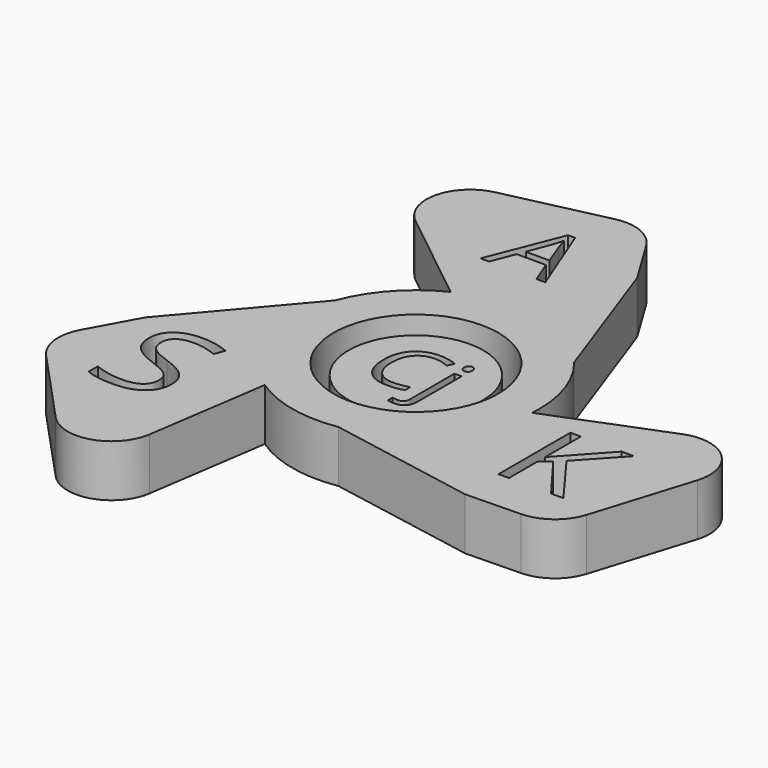
from build123d import *

# Parameters (mm, degrees)
F0_R          = 11.1
F1_DEPTH      = 7
F2_TEXT_SIZE  = 16.9441087766
F3_DEPTH      = 25.4
F4_TEXT_SIZE  = 13.7672423282
F5_DEPTH      = 25.4
F6_TEXT_SIZE  = 19.1516820431
F7_DEPTH      = 25.4
F8_R          = 9.0670245161
F9_DEPTH      = 5.588
F10_TEXT_SIZE = 11.9094963237
F11_DEPTH     = 25.4
F13_W         = 6
F13_H         = 1
F13_W_2       = 1
F13_H_2       = 3
F14_DEPTH     = 3


# Not quite as in the source:
# - Text() gives the source's letters only with a copy of the font that has no kerning and outlines rounded to 1/6400 em; it was checked with that copy


with BuildPart() as f1:
    # F0 (on Top) → F1 (new body)
    with BuildSketch(Plane.XY):
        with BuildLine():
            ThreePointArc((16.5940088671, -1.1747814046), (16.6251551137, -0.587757669), (16.635541519, 0))
            ThreePointArc((16.635541519, 0), (15.664947067, 5.5991673506), (12.8664216519, 10.5449720486))
            ThreePointArc((12.8664216519, 10.5449720486), (3.5598178716, 16.2501981019), (-7.2796138933, 14.9582239319))
            ThreePointArc((-7.2796138933, 14.9582239319), (-12.293175437, 11.2079917606), (-15.5654245023, 5.8701619821))
            ThreePointArc((-15.5654245023, 5.8701619821), (-15.8529933086, -5.0422063413), (-9.3143949738, -13.7834425273))
            ThreePointArc((-9.3143949738, -13.7834425273), (-3.5598178716, -16.2501981019), (2.6990028503, -16.4151340307))
            ThreePointArc((2.6990028503, -16.4151340307), (12.293175437, -11.2079917606), (16.5940088671, -1.1747814046))
        make_face()
        Circle(F0_R, mode=Mode.SUBTRACT)
        with BuildLine():
            ThreePointArc((-7.2796138933, 14.9582239319), (3.5598178716, 16.2501981019), (12.8664216519, 10.5449720486))
            Line((12.8664216519, 10.5449720486), (6.0360450298, 29.6823140234))
            Line((6.0360450298, 29.6823140234), (2.1992372512, 35.9986009481))
            ThreePointArc((2.1992372512, 35.9986009481), (-0.5333593719, 38.362277675), (-4.1319169388, 38.6854423552))
            Line((-4.1319169388, 38.6854423552), (-17.8556635882, 35.5845182616))
            ThreePointArc((-17.8556635882, 35.5845182616), (-22.2992502488, 31.1502452294), (-20.2187305905, 25.227435281))
            Line((-20.2187305905, 25.227435281), (-7.2796138933, 14.9582239319))
        make_face()
        with BuildLine():
            Line((31.9569651209, 4.8962166832), (16.5940088671, -1.1747814046))
            ThreePointArc((16.5940088671, -1.1747814046), (12.293175437, -11.2079917606), (2.6990028503, -16.4151340307))
            Line((2.6990028503, -16.4151340307), (22.6876154725, -20.0685253458))
            Line((22.6876154725, -20.0685253458), (30.0760842961, -19.9038958025))
            ThreePointArc((30.0760842961, -19.9038958025), (33.4893866995, -18.7192360721), (35.5685343057, -15.7643761422))
            Line((35.5685343057, -15.7643761422), (39.7449285901, -2.328800862))
            ThreePointArc((39.7449285901, -2.328800862), (38.1265288272, 3.7365945861), (31.9569651209, 4.8962166832))
        make_face()
        with BuildLine():
            ThreePointArc((-9.3143949738, -13.7834425273), (-15.8529933086, -5.0422063413), (-15.5654245023, 5.8701619821))
            Line((-15.5654245023, 5.8701619821), (-28.7236605022, -9.6137886775))
            Line((-28.7236605022, -9.6137886775), (-32.2753215473, -16.0947051456))
            ThreePointArc((-32.2753215473, -16.0947051456), (-32.9560273276, -19.6430416029), (-31.4366173668, -22.921066213))
            Line((-31.4366173668, -22.921066213), (-21.8892650019, -33.2557173997))
            ThreePointArc((-21.8892650019, -33.2557173997), (-15.8272785784, -34.8868398155), (-11.7382345304, -30.1236519642))
            Line((-11.7382345304, -30.1236519642), (-9.3143949738, -13.7834425273))
        make_face()
    extrude(amount=F1_DEPTH)

    # F2 (on face) → F3 (cut)
    with BuildSketch(Plane.XY.offset(7)):
        with Locations((20.8926647902, -14.2971209716)):
            Text('K', F2_TEXT_SIZE, font='Open Sans', text_align=(TextAlign.LEFT, TextAlign.BOTTOM))
    extrude(amount=-F3_DEPTH, mode=Mode.SUBTRACT)

    # F4 (on face) → F5 (cut)
    with BuildSketch(Plane.XY.offset(7)):
        with Locations((-9.6048026555, 22.8818524629)):
            Text('A', F4_TEXT_SIZE, font='Open Sans', text_align=(TextAlign.LEFT, TextAlign.BOTTOM))
    extrude(amount=-F5_DEPTH, mode=Mode.SUBTRACT)

    # F6 (on face) → F7 (cut)
    with BuildSketch(Plane.XY.offset(7)):
        with Locations((-26.6629411844, -23.4029997485)):
            Text('S', F6_TEXT_SIZE, font='Open Sans', text_align=(TextAlign.LEFT, TextAlign.BOTTOM))
    extrude(amount=-F7_DEPTH, mode=Mode.SUBTRACT)

    # F13 (on offset) → F14 (join)
    with BuildSketch(Plane.XY.offset(2)):
        with Locations((-5.2444588744, 29.0356876091)):
            Rectangle(F13_W, F13_H)
        with Locations((-5.2444588744, 26.5356876091)):
            Rectangle(F13_W_2, F13_H_2)
    extrude(amount=F14_DEPTH)


with BuildPart() as f9:
    # F8 (on Top) → F9 (new body)
    with BuildSketch(Plane.XY):
        Circle(F8_R)
    extrude(amount=F9_DEPTH)

    # F10 (on face) → F11 (cut)
    with BuildSketch(Plane.XY.offset(5.588)):
        with Locations((-5.5870884098, -3.5751680844)):
            Text('Cj', F10_TEXT_SIZE, font='Open Sans', text_align=(TextAlign.LEFT, TextAlign.BOTTOM))
    extrude(amount=-F11_DEPTH, mode=Mode.SUBTRACT)


solid = Compound([f1.part, f9.part])
